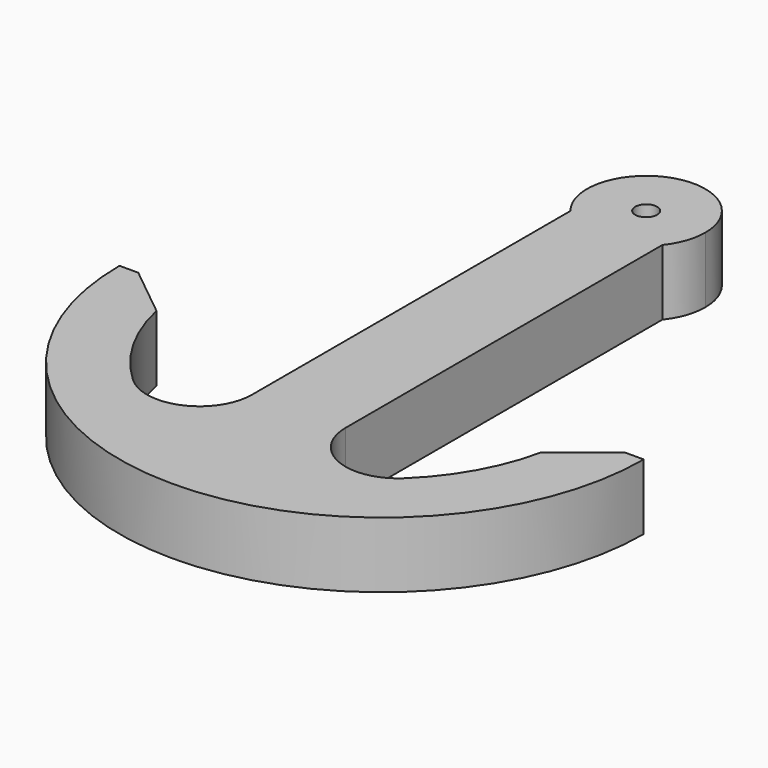
from build123d import *

# Parameters (mm, degrees)
F1_R        = 1.6666666667
F2_DEPTH    = 10
F3_T1_DEPTH = 46.985990025
F4_R        = 8


# Not quite as in the source:
# - a fillet or chamfer that OpenCascade refuses, or shapes differently, is made with other operations: its cross-section is extruded or revolved along the edge and cut away or added
# - a feature names something its author has since deleted; it is built from what else it names


with BuildPart() as f2:
    # F1 (on Top) → F2 (new body)
    with BuildSketch(Plane.XY):
        with BuildLine():
            ThreePointArc((7, 48.9616353347), (0, 52.3047810852), (-7, 48.9616353347))
            Line((-7, 48.9616353347), (7, 48.9616353347))
        make_face()
        with BuildLine():
            Line((7, 48.9616353347), (-7, 48.9616353347))
            Line((-7, 48.9616353347), (-7, 37.6479268357))
            ThreePointArc((-7, 37.6479268357), (0, 34.3047810852), (7, 37.6479268357))
            Line((7, 37.6479268357), (7, 48.9616353347))
        make_face()
        with Locations((0, 43.3047810852)):
            Circle(F1_R, mode=Mode.SUBTRACT)
        with BuildLine():
            Line((-7, 37.6479268357), (-7, 48.9616353347))
            ThreePointArc((-7, 48.9616353347), (-9, 43.3047810852), (-7, 37.6479268357))
        make_face()
        with BuildLine():
            ThreePointArc((9, 43.3047810852), (8.4852813742, 46.3047810852), (7, 48.9616353347))
            Line((7, 48.9616353347), (7, 37.6479268357))
            ThreePointArc((7, 37.6479268357), (8.4852813742, 40.3047810852), (9, 43.3047810852))
        make_face()
        with BuildLine():
            ThreePointArc((7, 37.6479268357), (0, 34.3047810852), (-7, 37.6479268357))
            Line((-7, 37.6479268357), (-7, -35.8969497675))
            ThreePointArc((-7, -35.8969497675), (0.0040151824, -36.6948708101), (7, -35.8293633875))
            Line((7, -35.8293633875), (7, 37.6479268357))
        make_face()
        with BuildLine():
            ThreePointArc((7, -35.8293633875), (0.0040151824, -36.6948708101), (-7, -35.8969497675))
            ThreePointArc((-7, -35.8969497675), (-23.5639927575, -25.3622297337), (-30.0136384001, -6.8217806199))
            Line((-30.0136384001, -6.8217806199), (-39.6402001052, -6.8217806199))
            Line((-39.6402001052, -6.8217806199), (-40.0136384001, -6.8217806199))
            ThreePointArc((-40.0136384001, -6.8217806199), (-0.1402001052, -46.6952189148), (39.7332381897, -6.8217806199))
            Line((39.7332381897, -6.8217806199), (29.7332381897, -6.8217806199))
            ThreePointArc((29.7332381897, -6.8217806199), (23.3728244006, -25.248934338), (7, -35.8293633875))
        make_face()
    extrude(amount=F2_DEPTH)

    # F3: chamfer of 8 on 2 edges, made by hand

    # F3_s2 → F3_t1 (cut)
    with BuildSketch(Plane.XY.offset(-18.4929950125)):
        with BuildLine():
            Line((-29.3395867315, -13.1319419656), (-37.1590781039, -6.8217806199))
            Line((-37.1590781039, -6.8217806199), (-30.0136384001, -6.8217806199))
            ThreePointArc((-30.0136384001, -6.8217806199), (-29.8322989719, -10.108356414), (-29.3395867315, -13.1319419656))
        make_face()
        with BuildLine():
            Line((36.8786778935, -6.8217806199), (29.0591865211, -13.1319419656))
            ThreePointArc((29.0591865211, -13.1319419656), (29.5518987615, -10.108356414), (29.7332381897, -6.8217806199))
            Line((29.7332381897, -6.8217806199), (36.8786778935, -6.8217806199))
        make_face()
    extrude(amount=F3_T1_DEPTH, mode=Mode.SUBTRACT)

    # F4
    f4_edges = [f2.edges().sort_by_distance(p)[0] for p in [
        (-7, -35.89695, 5),
        (7, -35.829363, 5),
    ]]
    fillet(f4_edges, radius=F4_R)


solid = f2.part
